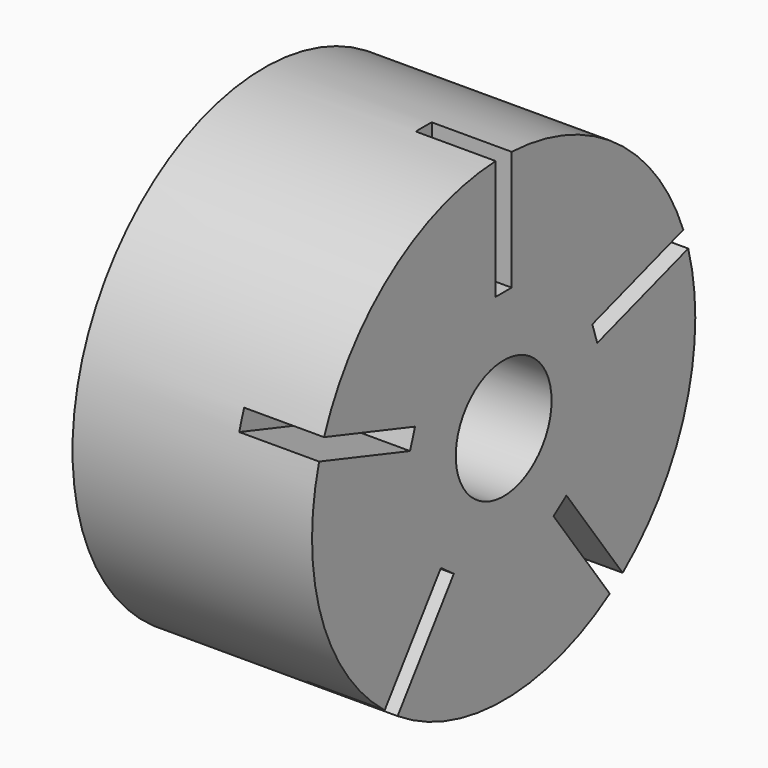
from build123d import *

# Parameters (mm, degrees)
F0_R            = 38.1
F1_DEPTH        = 38.1
F3_START        = 19.05
F2_W            = 12.7
F2_H            = 3.175
F3_DEPTH        = 19.05
F3_COPIES_COUNT = 5
F4_R            = 9.525
F5_DEPTH        = 38.101


# Not quite as in the source:
# - a pattern or mirror of a feature is missing from the dataset's text; its kind, count and spacing are read off the source's solid


with BuildPart() as f1:
    # F0 (on Right) → F1 (new body)
    with BuildSketch(Plane.YZ):
        Circle(F0_R)
    extrude(amount=F1_DEPTH)

    # F2 (on Top) → F3 (cut)
    with BuildSketch(Plane.XY.offset(F3_START)):
        with Locations((31.75, 0)):
            Rectangle(F2_W, F2_H)
    f3 = extrude(amount=F3_DEPTH, mode=Mode.SUBTRACT)

    # F3_copies: F3 ×5 about axis
    f3_copies_axis = Axis((0, 0, 0), (1, 0, 0))
    for i in range(1, F3_COPIES_COUNT):
        add(f3.rotate(f3_copies_axis, i * 360 / F3_COPIES_COUNT), mode=Mode.SUBTRACT)

    # F4 (on face) → F5 (cut, through all)
    with BuildSketch(Plane.YZ.offset(38.1)):
        Circle(F4_R)
    extrude(amount=-F5_DEPTH, mode=Mode.SUBTRACT)


solid = f1.part
